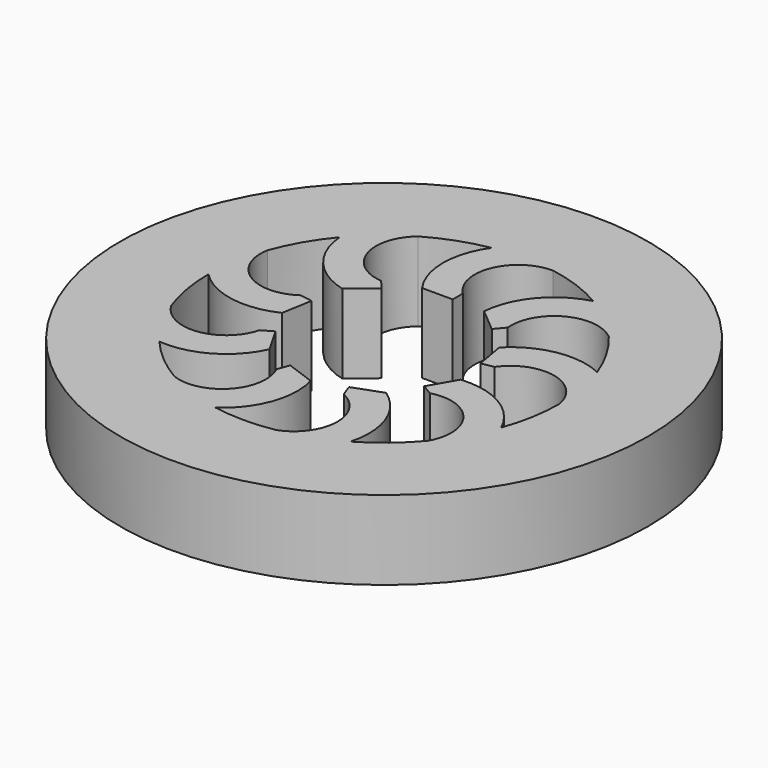
from build123d import *

# Parameters (mm, degrees)
F0_R            = 10
F0_R_2          = 6.65
F1_DEPTH        = 3
F3_DEPTH        = 3
F3_COPIES_COUNT = 9


# Not quite as in the source:
# - a pattern or mirror of a feature is missing from the dataset's text; its kind, count and spacing are read off the source's solid
# - a feature names something its author has since deleted; it is built from what else it names


with BuildPart() as f1:
    # F0 (on Top) → F1 (new body)
    with BuildSketch(Plane.XY):
        Circle(F0_R)
        Circle(F0_R_2, mode=Mode.SUBTRACT)
    extrude(amount=F1_DEPTH)

    # F2 (on Top) → F3 (join, through all)
    with BuildSketch(Plane.XY):
        with BuildLine():
            ThreePointArc((0, 3.7286332735), (-0.3629275105, 5.527055954), (1.161605891, 6.5477608199))
            ThreePointArc((1.161605891, 6.5477608199), (0, 6.65), (-1.161605891, 6.5477608199))
            ThreePointArc((-1.161605891, 6.5477608199), (-1.6872745189, 4.8988804099), (-1.161605891, 3.25))
            Line((-1.161605891, 3.25), (0, 3.25))
            Line((0, 3.25), (0, 3.7286332735))
        make_face()
    f3 = extrude(amount=F3_DEPTH)

    # F3_copies: F3 ×9 about axis
    f3_copies_axis = Axis((0, 0, 0), (0, 0, 1))
    for i in range(1, F3_COPIES_COUNT):
        add(f3.rotate(f3_copies_axis, i * 360 / F3_COPIES_COUNT))


solid = f1.part
